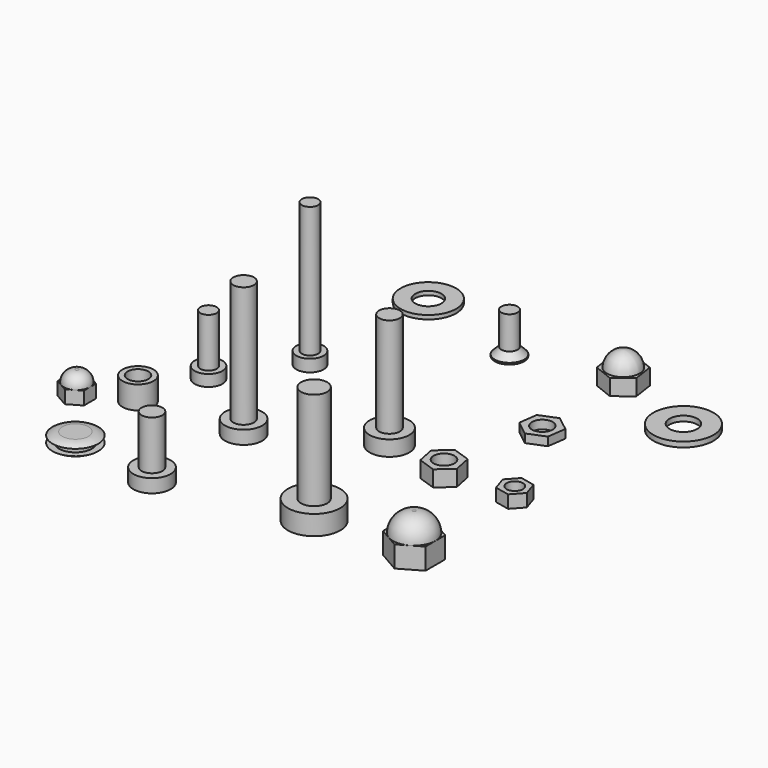
from build123d import *

# Parameters (mm, degrees)
F0_R      = 3.175
F1_DEPTH  = 30.5
F2_R      = 6.075
F3_DEPTH  = 4.7
F4_R      = 3.175
F5_DEPTH  = 4.9
F6_R      = 3.175
F7_DEPTH  = 37
F8_R      = 5.7
F9_DEPTH  = 4.1
F10_R     = 3.175
F11_DEPTH = 2.6
F12_R     = 2.5
F13_DEPTH = 3.9
F14_R     = 2.5
F15_DEPTH = 40
F16_R     = 4.15
F17_DEPTH = 3.7
F18_R     = 2.5
F19_DEPTH = 15
F20_R     = 4.25
F21_DEPTH = 3.5
F22_R     = 3.175
F23_DEPTH = 4.9
F24_R     = 5
F25_DEPTH = 4.8
F27_R     = 5
F27_R_2   = 4
F28_DEPTH = 1
F29_R     = 7
F30_DEPTH = 1
F32_R     = 7
F32_R_2   = 4
F33_DEPTH = 1
F35_R     = 4
F36_DEPTH = 30
F37_R     = 8
F38_DEPTH = 6
F39_R     = 4
F40_DEPTH = 6.5
F41_R     = 6.5
F42_DEPTH = 6
F43_R     = 5.99999
F44_R     = 8.5
F44_R_2   = 4
F45_DEPTH = 1.2
F46_R     = 4.75
F46_R_2   = 3.175
F47_DEPTH = 7
F48_R     = 3.175
F49_DEPTH = 15
F50_R     = 5.7
F51_DEPTH = 4.1
F52_R     = 9.2
F52_R_2   = 4.25
F53_DEPTH = 1.6
F54_R     = 2.5
F55_DEPTH = 4
F56_R     = 4
F57_DEPTH = 3.5
F58_R     = 3.49999
F59_R     = 2.5
F60_DEPTH = 10
F61_R     = 4.5
F62_DEPTH = 2.5
F63_SIZE  = 1.99999


# Not quite as in the source:
# - a fillet or chamfer that OpenCascade refuses, or shapes differently, is made with other operations: its cross-section is extruded or revolved along the edge and cut away or added
# - a fillet or chamfer is up to 0.001 mm smaller than in the source, because OpenCascade refuses the exact size


with BuildPart() as f1:
    # F0 (on Top) → F1 (new body)
    with BuildSketch(Plane.XY):
        Circle(F0_R)
    extrude(amount=F1_DEPTH)

    # F2 (on face) → F3 (join)
    with BuildSketch(Plane(origin=(0, 0, 0), x_dir=(1, 0, 0), z_dir=(0, 0, -1))):
        Circle(F2_R)
    extrude(amount=F3_DEPTH)


with BuildPart() as f5:
    # F4 (on Top) → F5 (new body)
    with BuildSketch(Plane.XY):
        Polygon((25.2304555405, -6.5690084936), (20.9913269575, -10.3164238949), (22.117119602, -15.8613246384), (27.4820408295, -17.6588099806), (31.7211694126, -13.9113945793), (30.5953767681, -8.3664938358), align=None)
        with Locations((26.356248185, -12.1139092371)):
            Circle(F4_R, mode=Mode.SUBTRACT)
    extrude(amount=F5_DEPTH)


with BuildPart() as f7:
    # F6 (on Top) → F7 (new body)
    with BuildSketch(Plane.XY):
        with Locations((-30.0902538002, -18.1267801672)):
            Circle(F6_R)
    extrude(amount=F7_DEPTH)

    # F8 (on face) → F9 (join)
    with BuildSketch(Plane(origin=(0, 0, 0), x_dir=(1, 0, 0), z_dir=(0, 0, -1))):
        with Locations((-30.0902538002, 18.1267801672)):
            Circle(F8_R)
    extrude(amount=F9_DEPTH)


with BuildPart() as f11:
    # F10 (on Top) → F11 (new body)
    with BuildSketch(Plane.XY):
        Polygon((36.3389975742, 21.8056498979), (31.810116069, 25.3397785947), (26.4850300848, 23.1847165088), (25.6888256057, 17.4955257262), (30.2177071109, 13.9613970295), (35.5427930952, 16.1164591153), align=None)
        with Locations((31.01391159, 19.6505878121)):
            Circle(F10_R, mode=Mode.SUBTRACT)
    extrude(amount=F11_DEPTH)


with BuildPart() as f13:
    # F12 (on Top) → F13 (new body)
    with BuildSketch(Plane.XY):
        Polygon((49.9805748483, -7.4299281605), (45.5503371745, -6.4739849159), (42.5073472032, -9.8327116639), (43.8945949057, -14.1473816565), (48.3248325795, -15.1033249012), (51.3678225508, -11.7445981532), align=None)
        with Locations((46.937584877, -10.7886549085)):
            Circle(F12_R, mode=Mode.SUBTRACT)
    extrude(amount=F13_DEPTH)


with BuildPart() as f15:
    # F14 (on Top) → F15 (new body)
    with BuildSketch(Plane.XY):
        with Locations((-39.6681278944, 19.2128680646)):
            Circle(F14_R)
    extrude(amount=F15_DEPTH)

    # F16 (on face) → F17 (join)
    with BuildSketch(Plane(origin=(0, 0, 0), x_dir=(1, 0, 0), z_dir=(0, 0, -1))):
        with Locations((-39.6681278944, -19.2128680646)):
            Circle(F16_R)
    extrude(amount=F17_DEPTH)


with BuildPart() as f19:
    # F18 (on Top) → F19 (new body)
    with BuildSketch(Plane.XY):
        with Locations((-53.7162348628, -2.0106609445)):
            Circle(F18_R)
    extrude(amount=F19_DEPTH)

    # F20 (on face) → F21 (join)
    with BuildSketch(Plane(origin=(0, 0, 0), x_dir=(1, 0, 0), z_dir=(0, 0, -1))):
        with Locations((-53.7162348628, 2.0106609445)):
            Circle(F20_R)
    extrude(amount=F21_DEPTH)


with BuildPart() as f23:
    # F22 (on Top) → F23 (new body)
    with BuildSketch(Plane.XY):
        Polygon((29.1114152461, 58.0769082309), (24.1508137011, 54.1577332779), (25.0646179998, 47.9021388454), (30.9390238435, 45.5657193659), (35.8996253884, 49.484894319), (34.9858210897, 55.7404887514), align=None)
        with Locations((30.0252195448, 51.8213137984)):
            Circle(F22_R, mode=Mode.SUBTRACT)
    extrude(amount=F23_DEPTH)

    # F24 (on face) → F25 (join)
    with BuildSketch(Plane.XY.offset(4.9)):
        with Locations((30.0252195448, 51.8213137984)):
            Circle(F24_R)
    extrude(amount=F25_DEPTH)

    # F26: fillet of radius 5 on 1 edges, made by hand

    # F26_s1 → F26_t2 (revolve, cut)
    with BuildSketch(Plane.XZ.offset(-51.8213137984)):
        with BuildLine():
            ThreePointArc((35.0252195448, 4.9), (33.4933227612, 8.3055512755), (30.029221146, 9.7))
            Line((30.029221146, 9.7), (35.0252195448, 9.7))
            Line((35.0252195448, 9.7), (35.0252195448, 4.9))
        make_face()
    revolve(axis=Axis((30.0252195448, 51.8213137984, 9.7), (0, 0, 1)), mode=Mode.SUBTRACT)


with BuildPart() as f28:
    # F27 (on Top) → F28 (new body, symmetric)
    with BuildSketch(Plane.XY):
        with Locations((-54.8807457089, -51.4248013496)):
            Circle(F27_R)
        with Locations((-54.8807457089, -51.4248013496)):
            Circle(F27_R_2, mode=Mode.SUBTRACT)
    extrude(amount=F28_DEPTH, both=True)

    # F29 (on face) → F30 (join)
    with BuildSketch(Plane.XY.offset(1)):
        with Locations((-54.8807457089, -51.4248013496)):
            Circle(F29_R)
    extrude(amount=F30_DEPTH)

    # F31: fillet of radius 5 on 1 edges, made by hand

    # F31_s1 → F31_t2 (revolve, cut)
    with BuildSketch(Plane.XZ.offset(51.4248013496)):
        with BuildLine():
            ThreePointArc((-47.8807457089, 1), (-49.2996068789, 1.7434164903), (-50.8807457089, 2))
            Line((-50.8807457089, 2), (-47.8807457089, 2))
            Line((-47.8807457089, 2), (-47.8807457089, 1))
        make_face()
    revolve(axis=Axis((-54.8807457089, -51.4248013496, 2), (0, 0, 1)), mode=Mode.SUBTRACT)

    # F32 (on face) → F33 (join)
    with BuildSketch(Plane(origin=(0, 0, -1), x_dir=(1, 0, 0), z_dir=(0, 0, -1))):
        with Locations((-54.8807457089, 51.4248013496)):
            Circle(F32_R)
        with Locations((-54.8807457089, 51.4248013496)):
            Circle(F32_R_2, mode=Mode.SUBTRACT)
    extrude(amount=F33_DEPTH)

    # F34: fillet of radius 5 on 1 edges, made by hand

    # F34_s1 → F34_t2 (revolve, cut)
    with BuildSketch(Plane.XZ.offset(51.4248013496)):
        with BuildLine():
            ThreePointArc((-47.8807457089, -1), (-49.2996068789, -1.7434164903), (-50.8807457089, -2))
            Line((-50.8807457089, -2), (-47.8807457089, -2))
            Line((-47.8807457089, -2), (-47.8807457089, -1))
        make_face()
    revolve(axis=Axis((-54.8807457089, -51.4248013496, -2), (0, 0, -1)), mode=Mode.SUBTRACT)


with BuildPart() as f36:
    # F35 (on Top) → F36 (new body)
    with BuildSketch(Plane.XY):
        with Locations((8.8167153299, -39.8334674537)):
            Circle(F35_R)
    extrude(amount=F36_DEPTH)

    # F37 (on face) → F38 (join)
    with BuildSketch(Plane(origin=(0, 0, 0), x_dir=(1, 0, 0), z_dir=(0, 0, -1))):
        with Locations((8.8167153299, 39.8334674537)):
            Circle(F37_R)
    extrude(amount=F38_DEPTH)


with BuildPart() as f40:
    # F39 (on Top) → F40 (new body)
    with BuildSketch(Plane.XY):
        Polygon((39.9360788465, -44.8762761873), (39.9360788465, -52.3818296868), (46.4360788465, -56.1346064365), (52.9360788465, -52.3818296868), (52.9360788465, -44.8762761873), (46.4360788465, -41.1234994376), align=None)
        with Locations((46.4360788465, -48.629052937)):
            Circle(F39_R, mode=Mode.SUBTRACT)
    extrude(amount=F40_DEPTH)

    # F41 (on face) → F42 (join)
    with BuildSketch(Plane.XY.offset(6.5)):
        with Locations((46.4360788465, -48.629052937)):
            Circle(F41_R)
    extrude(amount=F42_DEPTH)

    # F43 (radius 6 in the source; OpenCascade refuses exactly that, so slightly less here)
    f43_edges = [f40.edges().sort_by_distance(p)[0] for p in [
        (39.936079, -48.629053, 12.5),
    ]]
    fillet(f43_edges, radius=F43_R)


with BuildPart() as f45:
    # F44 (on Top) → F45 (new body)
    with BuildSketch(Plane.XY):
        with Locations((-32.9999290407, 56.1005584896)):
            Circle(F44_R)
        with Locations((-32.9999290407, 56.1005584896)):
            Circle(F44_R_2, mode=Mode.SUBTRACT)
    extrude(amount=F45_DEPTH)


with BuildPart() as f47:
    # F46 (on Top) → F47 (new body)
    with BuildSketch(Plane.XY):
        with Locations((-55.4018653929, -26.8562659621)):
            Circle(F46_R)
        with Locations((-55.4018653929, -26.8562659621)):
            Circle(F46_R_2, mode=Mode.SUBTRACT)
    extrude(amount=F47_DEPTH)


with BuildPart() as f49:
    # F48 (on Top) → F49 (new body)
    with BuildSketch(Plane.XY):
        with Locations((-31.514249742, -51.3591133058)):
            Circle(F48_R)
    extrude(amount=F49_DEPTH)

    # F50 (on face) → F51 (join)
    with BuildSketch(Plane(origin=(0, 0, 0), x_dir=(1, 0, 0), z_dir=(0, 0, -1))):
        with Locations((-31.514249742, 51.3591133058)):
            Circle(F50_R)
    extrude(amount=F51_DEPTH)


with BuildPart() as f53:
    # F52 (on Top) → F53 (new body)
    with BuildSketch(Plane.XY):
        with Locations((55.4715134203, 43.0044569075)):
            Circle(F52_R)
        with Locations((55.4715134203, 43.0044569075)):
            Circle(F52_R_2, mode=Mode.SUBTRACT)
    extrude(amount=F53_DEPTH)


with BuildPart() as f55:
    # F54 (on Top) → F55 (new body)
    with BuildSketch(Plane.XY):
        Polygon((-72.1124851108, -32.018936682), (-72.1124851108, -36.6377388355), (-68.1124851108, -38.9471399123), (-64.1124851108, -36.6377388355), (-64.1124851108, -32.018936682), (-68.1124851108, -29.7095356053), align=None)
        with Locations((-68.1124851108, -34.3283377588)):
            Circle(F54_R, mode=Mode.SUBTRACT)
    extrude(amount=F55_DEPTH)

    # F56 (on face) → F57 (join)
    with BuildSketch(Plane.XY.offset(4)):
        with Locations((-68.1124851108, -34.3283377588)):
            Circle(F56_R)
    extrude(amount=F57_DEPTH)

    # F58 (radius 3.5 in the source; OpenCascade refuses exactly that, so slightly less here)
    f58_edges = [f55.edges().sort_by_distance(p)[0] for p in [
        (-72.112485, -34.328338, 7.5),
    ]]
    fillet(f58_edges, radius=F58_R)


with BuildPart() as f60:
    # F59 (on Top) → F60 (new body)
    with BuildSketch(Plane.XY):
        with Locations((-3.7879089359, 50.5888238549)):
            Circle(F59_R)
    extrude(amount=F60_DEPTH)

    # F61 (on face) → F62 (join)
    with BuildSketch(Plane(origin=(0, 0, 0), x_dir=(1, 0, 0), z_dir=(0, 0, -1))):
        with Locations((-3.7879089359, -50.5888238549)):
            Circle(F61_R)
    extrude(amount=F62_DEPTH)

    # F63 (size 2 in the source; OpenCascade refuses exactly that, so slightly less here)
    f63_edges = [f60.edges().sort_by_distance(p)[0] for p in [
        (-8.287909, 50.588824, 0),
    ]]
    chamfer(f63_edges, length=F63_SIZE)


solid = Compound([f1.part, f5.part, f7.part, f11.part, f13.part, f15.part, f19.part, f23.part, f28.part, f36.part, f40.part, f45.part, f47.part, f49.part, f53.part, f55.part, f60.part])
